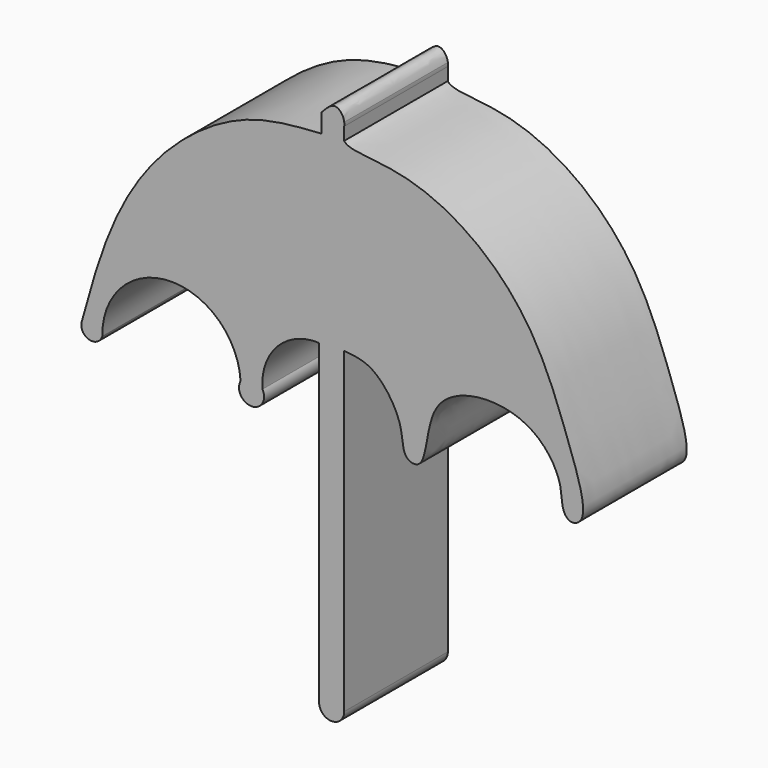
from build123d import *

# Parameters (mm, degrees)
F1_DEPTH = 6.35


with BuildPart() as f1:
    # F0 (on Front) → F1 (new body)
    with BuildSketch(Plane.XZ):
        with BuildLine():
            add(Edge.make_bspline(
                [(-12.4509278685, -0.6481549935), (-12.0317981163, 0.8810850321), (-11.1928806268, 3.9419658126), (-8.7731819463, 8.0717111222), (-4.6589539948, 11.0646575395), (-1.9667442238, 11.2383011146), (-0.6972711999, 11.3201802596)],
                knots=[0, 0, 0, 0, 0.2552710683, 0.5109428826, 0.7693921089, 1, 1, 1, 1], degree=3))
            ThreePointArc((-12.4509278685, -0.6481549935), (-12.0714345726, -1.2777296563), (-11.4312041551, -0.9165033698))
            ThreePointArc((-11.4312041551, -0.9165033698), (-8.1735331436, 2.540236173), (-4.6527902596, -0.6481549935))
            ThreePointArc((-4.6527902596, -0.6481549935), (-4.1167481077, -1.5631866704), (-3.5767615773, -0.65047713))
            ThreePointArc((-3.5767615773, -0.65047713), (-2.8498328125, 1.4297474764), (-0.8046104922, 2.2500068881))
            Line((-0.8046104922, 2.2500068881), (-0.8046104922, -13.2605265826))
            ThreePointArc((-0.8046104922, -13.2605265826), (-0.1874094887, -13.8777275861), (0.4297915148, -13.2605265826))
            Line((0.4297915148, -13.2605265826), (0.4297915148, 2.3036766797))
            add(Edge.make_bspline(
                [(0.4297915148, 11.3738495857), (0.6526590266, 11.0354959137), (3.1750938666, 11.1025792799), (6.7730940941, 9.5016063693), (9.8367590632, 6.2932480095), (11.3370440892, 2.2324782786), (12.5111170003, -1.1337690095), (11.4960734497, -1.6007523467), (11.0548187099, -0.9951418024), (11.1366100355, 0.0760910817), (10.0928611655, 1.858972596), (7.6732235172, 2.7806239453), (4.3454002919, 1.8654920892), (4.560083764, -1.648726748), (3.221032359, -1.3835064308), (3.3910248353, 0.1096392917), (1.9671173501, 2.1836191556), (0.899214588, 2.2670170656), (0.4297915148, 2.3036766797)],
                knots=[0.1025391075, 0.1025391075, 0.1025391075, 0.1025391075, 0.1626708527, 0.2414465269, 0.3216670559, 0.4050734358, 0.4735549353, 0.5041965823, 0.5334513595, 0.5728818213, 0.6263024965, 0.6876981158, 0.7540154426, 0.8182473727, 0.849383834, 0.8940797423, 0.9534401308, 1, 1, 1, 1], degree=3))
            add(Edge.make_bspline(
                [(0.4297915148, 12.0000571072), (0.4090063726, 11.7638984672), (0.3270478417, 11.5298332853), (0.4297915148, 11.3738495857)],
                knots=[0.0748179008, 0.0748179008, 0.0748179008, 0.0748179008, 0.1025391075, 0.1025391075, 0.1025391075, 0.1025391075], degree=3))
            Line((0.4297915148, 12.0000571072), (0.4297915148, 12.1788950637))
            add(Edge.make_bspline(
                [(-0.6972711999, 12.232565321), (-0.4617125379, 12.4859727505), (-0.0140726245, 12.9675312669), (0.3996041066, 12.448062951), (0.4297915148, 12.1788950637)],
                knots=[0, 0, 0, 0, 0.0356714562, 0.0677876477, 0.0677876477, 0.0677876477, 0.0677876477], degree=3))
            Line((-0.6972711999, 12.232565321), (-0.6972711999, 11.3201802596))
        make_face()
        with BuildLine():
            add(Edge.make_bspline(
                [(-4.6527902596, 2.2500068881), (-4.6881874921, 3.0714366785), (-4.7572235022, 4.6734894757), (-4.2725077694, 6.7651050781), (-3.8302798792, 8.624568161), (-2.9833358257, 9.3901871644), (-2.6203936393, 9.9507790211), (-2.4440996349, 10.2230785415)],
                knots=[0, 0, 0, 0, 0.2423030576, 0.4725690445, 0.6839878774, 0.8465016065, 1, 1, 1, 1], degree=3))
            ThreePointArc((-4.6527902596, 2.2500068881), (-7.512749867, 3.504606312), (-10.5426330119, 2.7475086972))
            add(Edge.make_bspline(
                [(-2.4440996349, 10.2230785415), (-3.0070766004, 10.1316858633), (-4.257690828, 9.9286633763), (-6.7376812556, 8.6628460438), (-8.7407318384, 6.5446693266), (-9.9049465269, 4.091310483), (-10.5426330119, 2.7475086972)],
                knots=[0, 0, 0, 0, 0.1991808283, 0.442466376, 0.6946167571, 1, 1, 1, 1], degree=3))
        make_face(mode=Mode.SUBTRACT)
        with BuildLine():
            add(Edge.make_bspline(
                [(-0.1412717829, 10.4595618322), (0.1250668674, 10.4148679988), (0.6860593829, 10.3207288041), (1.4339723073, 9.5420411919), (2.0176690385, 9.2792735551), (2.7849622808, 7.8675029191), (3.2129807692, 6.8552668878), (3.426070787, 5.5098999096), (3.5684033089, 3.2815882405), (3.4437081145, 2.3401855324), (3.3891098574, 1.9279888365)],
                knots=[0, 0, 0, 0, 0.10280599, 0.2165415756, 0.3074449242, 0.4471391252, 0.567356297, 0.6988234719, 0.868128731, 1, 1, 1, 1], degree=3))
            ThreePointArc((3.3891098574, 1.9279888365), (-0.1504588872, 3.371185766), (-3.6900276318, 1.9279888365))
            add(Edge.make_bspline(
                [(-0.1412717829, 10.4595618322), (-0.482391014, 10.3318500079), (-1.1763661999, 10.0720322404), (-2.034374878, 9.2356141659), (-2.7630920424, 8.3498824032), (-3.2130686106, 7.0082514597), (-3.7058453302, 5.8544228935), (-3.8051869716, 2.8456866579), (-3.7203032002, 2.1692530116), (-3.6900276318, 1.9279888365)],
                knots=[0, 0, 0, 0, 0.1276600513, 0.2597124399, 0.3909770246, 0.5317726453, 0.6738447952, 0.8836699404, 1, 1, 1, 1], degree=3))
        make_face(mode=Mode.SUBTRACT)
        with BuildLine():
            add(Edge.make_bspline(
                [(2.1224920638, 10.2230785415), (2.4304280303, 10.2765295315), (3.2266466532, 10.4147357766), (5.6068331787, 9.0279478535), (6.8826619925, 8.1843022652), (8.574542946, 6.2175447591), (9.7061171069, 4.1431701929), (9.9614117746, 3.1688551838), (10.0718149915, 2.7475086972)],
                knots=[0, 0, 0, 0, 0.1239955817, 0.3206107828, 0.4761099998, 0.6691251888, 0.8569118428, 1, 1, 1, 1], degree=3))
            ThreePointArc((10.0718149915, 2.7475086972), (7.267371932, 3.4391746522), (4.6350378543, 2.2500068881))
            add(Edge.make_bspline(
                [(4.6350378543, 2.2500068881), (4.6713806841, 2.9541300324), (4.7473255067, 4.4255208857), (4.1589573729, 6.921382003), (3.5565525979, 8.9681272577), (2.5902403363, 9.8137504266), (2.1224920638, 10.2230785415)],
                knots=[0, 0, 0, 0, 0.2503331616, 0.5231157749, 0.769161811, 1, 1, 1, 1], degree=3))
        make_face(mode=Mode.SUBTRACT)
        with BuildLine():
            add(Edge.make_bspline(
                [(0.4297915148, 12.1788950637), (0.4363995561, 12.1199740551), (0.4350627431, 12.0599482599), (0.4297915148, 12.0000571072)],
                knots=[0.0677876477, 0.0677876477, 0.0677876477, 0.0677876477, 0.0748179008, 0.0748179008, 0.0748179008, 0.0748179008], degree=3))
            Line((0.4297915148, 12.1788950637), (0.4297915148, 12.0000571072))
        make_face()
        with BuildLine():
            Line((0.4297915148, 11.3738495857), (0.4297915148, 12.0000571072))
            add(Edge.make_bspline(
                [(0.4297915148, 12.0000571072), (0.4090063726, 11.7638984672), (0.3270478417, 11.5298332853), (0.4297915148, 11.3738495857)],
                knots=[0.0748179008, 0.0748179008, 0.0748179008, 0.0748179008, 0.1025391075, 0.1025391075, 0.1025391075, 0.1025391075], degree=3))
        make_face()
        with BuildLine():
            ThreePointArc((-10.5426330119, 2.7475086972), (-7.512749867, 3.504606312), (-4.6527902596, 2.2500068881))
            add(Edge.make_bspline(
                [(-4.6527902596, 2.2500068881), (-4.6881874921, 3.0714366785), (-4.7572235022, 4.6734894757), (-4.2725077694, 6.7651050781), (-3.8302798792, 8.624568161), (-2.9833358257, 9.3901871644), (-2.6203936393, 9.9507790211), (-2.4440996349, 10.2230785415)],
                knots=[0, 0, 0, 0, 0.2423030576, 0.4725690445, 0.6839878774, 0.8465016065, 1, 1, 1, 1], degree=3))
            add(Edge.make_bspline(
                [(-2.4440996349, 10.2230785415), (-3.0070766004, 10.1316858633), (-4.257690828, 9.9286633763), (-6.7376812556, 8.6628460438), (-8.7407318384, 6.5446693266), (-9.9049465269, 4.091310483), (-10.5426330119, 2.7475086972)],
                knots=[0, 0, 0, 0, 0.1991808283, 0.442466376, 0.6946167571, 1, 1, 1, 1], degree=3))
        make_face()
        with BuildLine():
            ThreePointArc((-3.6900276318, 1.9279888365), (-0.1504588872, 3.371185766), (3.3891098574, 1.9279888365))
            add(Edge.make_bspline(
                [(-0.1412717829, 10.4595618322), (0.1250668674, 10.4148679988), (0.6860593829, 10.3207288041), (1.4339723073, 9.5420411919), (2.0176690385, 9.2792735551), (2.7849622808, 7.8675029191), (3.2129807692, 6.8552668878), (3.426070787, 5.5098999096), (3.5684033089, 3.2815882405), (3.4437081145, 2.3401855324), (3.3891098574, 1.9279888365)],
                knots=[0, 0, 0, 0, 0.10280599, 0.2165415756, 0.3074449242, 0.4471391252, 0.567356297, 0.6988234719, 0.868128731, 1, 1, 1, 1], degree=3))
            add(Edge.make_bspline(
                [(-0.1412717829, 10.4595618322), (-0.482391014, 10.3318500079), (-1.1763661999, 10.0720322404), (-2.034374878, 9.2356141659), (-2.7630920424, 8.3498824032), (-3.2130686106, 7.0082514597), (-3.7058453302, 5.8544228935), (-3.8051869716, 2.8456866579), (-3.7203032002, 2.1692530116), (-3.6900276318, 1.9279888365)],
                knots=[0, 0, 0, 0, 0.1276600513, 0.2597124399, 0.3909770246, 0.5317726453, 0.6738447952, 0.8836699404, 1, 1, 1, 1], degree=3))
        make_face()
        with BuildLine():
            ThreePointArc((4.6350378543, 2.2500068881), (7.267371932, 3.4391746522), (10.0718149915, 2.7475086972))
            add(Edge.make_bspline(
                [(2.1224920638, 10.2230785415), (2.4304280303, 10.2765295315), (3.2266466532, 10.4147357766), (5.6068331787, 9.0279478535), (6.8826619925, 8.1843022652), (8.574542946, 6.2175447591), (9.7061171069, 4.1431701929), (9.9614117746, 3.1688551838), (10.0718149915, 2.7475086972)],
                knots=[0, 0, 0, 0, 0.1239955817, 0.3206107828, 0.4761099998, 0.6691251888, 0.8569118428, 1, 1, 1, 1], degree=3))
            add(Edge.make_bspline(
                [(4.6350378543, 2.2500068881), (4.6713806841, 2.9541300324), (4.7473255067, 4.4255208857), (4.1589573729, 6.921382003), (3.5565525979, 8.9681272577), (2.5902403363, 9.8137504266), (2.1224920638, 10.2230785415)],
                knots=[0, 0, 0, 0, 0.2503331616, 0.5231157749, 0.769161811, 1, 1, 1, 1], degree=3))
        make_face()
    extrude(amount=F1_DEPTH)


solid = f1.part
